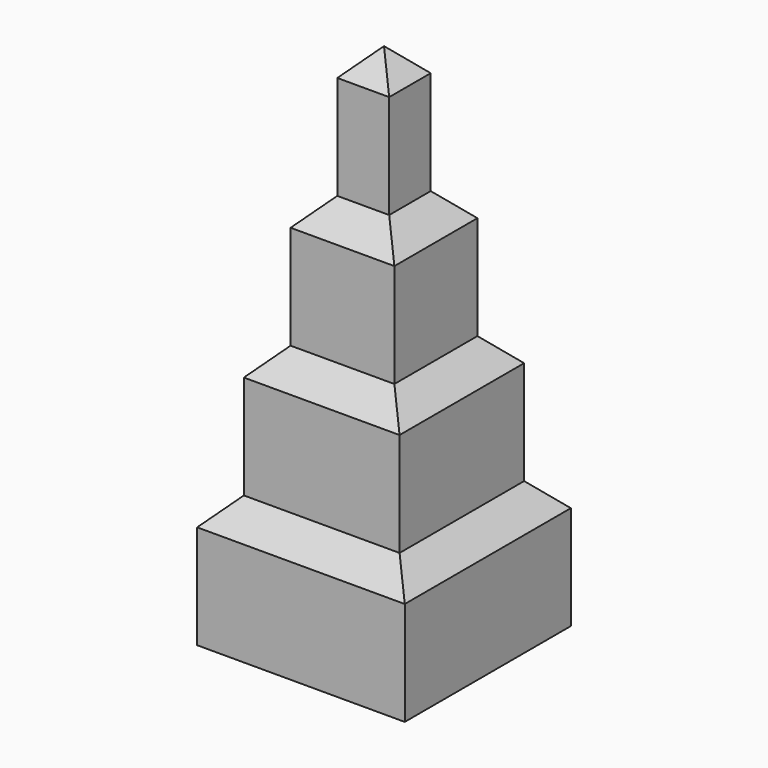
from build123d import *

# Parameters (mm, degrees)
F0_W     = 8
F0_H     = 8
F0_W_2   = 6
F0_H_2   = 6
F1_DEPTH = 5
F0_W_3   = 4
F0_H_3   = 4
F2_DEPTH = 10
F0_W_4   = 2
F0_H_4   = 2
F3_DEPTH = 15
F4_DEPTH = 20
F5_SIZE  = 0.99999


# Not quite as in the source:
# - a fillet or chamfer is up to 0.001 mm smaller than in the source, because OpenCascade refuses the exact size


with BuildPart() as f1:
    # F0 (on Top) → F1 (new body)
    with BuildSketch(Plane.XY):
        Rectangle(F0_W, F0_H)
        Rectangle(F0_W_2, F0_H_2, mode=Mode.SUBTRACT)
    extrude(amount=F1_DEPTH)

    # F0 (on Top) → F2 (join)
    with BuildSketch(Plane.XY):
        Rectangle(F0_W_2, F0_H_2)
        Rectangle(F0_W_3, F0_H_3, mode=Mode.SUBTRACT)
    extrude(amount=F2_DEPTH)

    # F0 (on Top) → F3 (join)
    with BuildSketch(Plane.XY):
        Rectangle(F0_W_3, F0_H_3)
        Rectangle(F0_W_4, F0_H_4, mode=Mode.SUBTRACT)
    extrude(amount=F3_DEPTH)

    # F0 (on Top) → F4 (join)
    with BuildSketch(Plane.XY):
        Rectangle(F0_W_4, F0_H_4)
    extrude(amount=F4_DEPTH)

    # F5 (size 1 in the source; OpenCascade refuses exactly that, so slightly less here)
    f5_edges = [f1.edges().sort_by_distance(p)[0] for p in [
        (0, -4, 5),
        (4, 0, 5),
        (0, 4, 5),
        (-4, 0, 5),
        (0, -3, 10),
        (3, 0, 10),
        (-3, 0, 10),
        (0, 3, 10),
        (2, 0, 15),
        (0, -2, 15),
        (-2, 0, 15),
        (0, 2, 15),
        (1, 0, 20),
        (0, -1, 20),
        (-1, 0, 20),
        (0, 1, 20),
    ]]
    chamfer(f5_edges, length=F5_SIZE)


solid = f1.part
